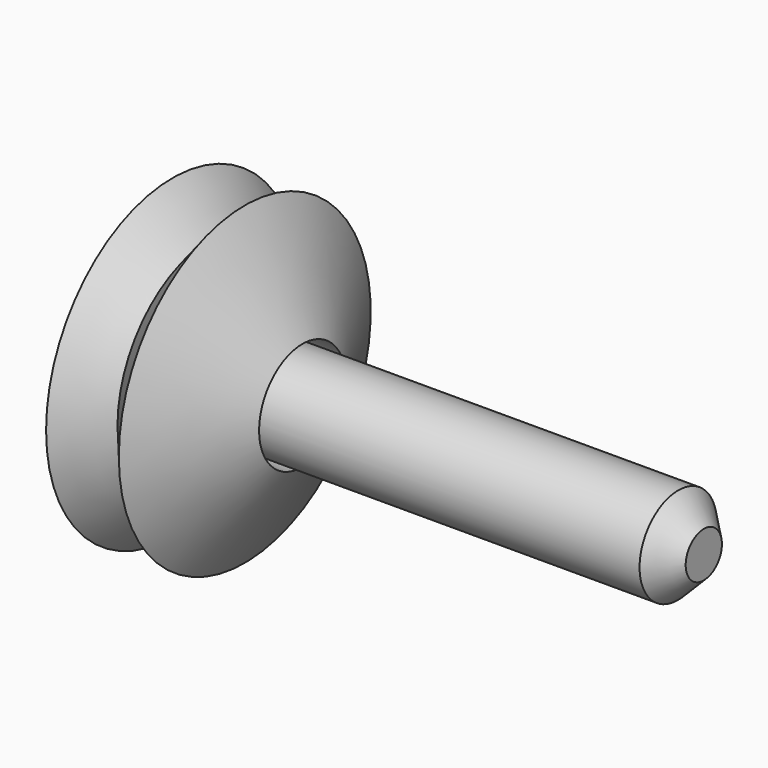
from build123d import *

# Parameters (mm, degrees)
F2_R     = 6.2211982037
F3_DEPTH = 19.1516
F4_DEPTH = 55.372
F5_SIZE  = 3.302


# Not quite as in the source:
# - the program builds the solid bodies; features that only make, move or delete a surface that nothing else refers to are left out


with BuildPart() as f1:
    # F0 (on Top) → F1 (revolve)
    with BuildSketch(Plane.XY):
        Polygon((-17.0599853833, 6.2996733477), (-20.4250291926, 4.9693077386), (-13.2254017106, -8.4908647026), (-8.2169655835, -3.2476578449), (-3.9128408491, -8.4126079255), (3.521556964, 4.8910505621), (-2.2694479322, 4.8910505621), (-5.1649496812, 0), (-8.2952223605, 2.6998602059), (-12.2546622766, -1.8907947353), align=None)
    revolve(axis=Axis((-9.930120464, 11.8798027962, 0), (1, 0, 0)))

    # F2 (on Right) → F3 (join)
    with BuildSketch(Plane.YZ):
        with Locations((11.7291258648, 0)):
            Circle(F2_R)
    extrude(amount=-F3_DEPTH)

    # F4 (add): a face of the model
    f4_faces = [f1.faces().sort_by_distance(p)[0] for p in [
        (0, 11.7291258648, 0),
    ]]
    extrude(f4_faces, amount=F4_DEPTH)

    # F5
    f5_edges = [f1.edges().sort_by_distance(p)[0] for p in [
        (55.372, 5.507928, 0),
    ]]
    chamfer(f5_edges, length=F5_SIZE)


solid = f1.part
